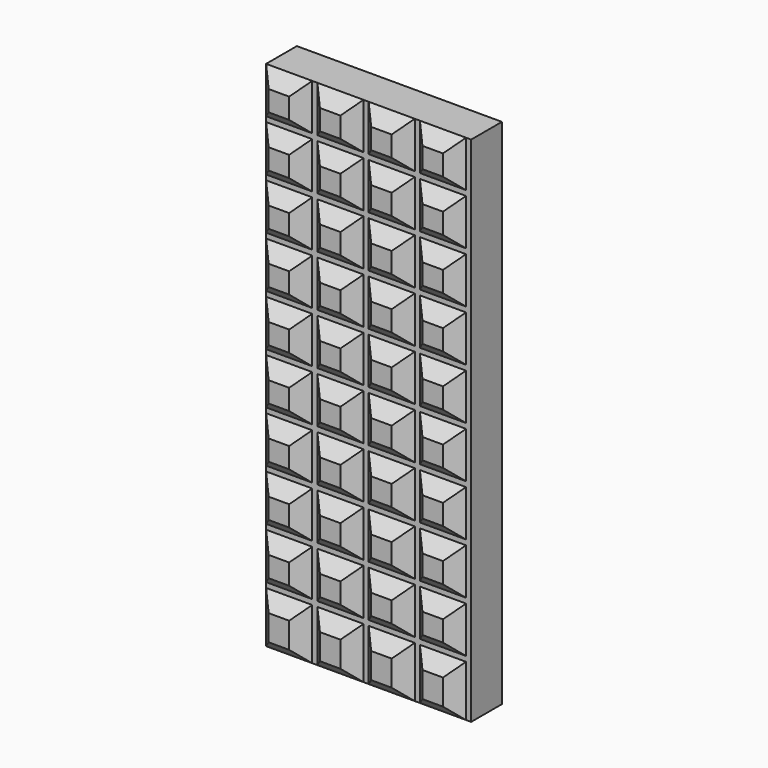
from build123d import *

# Parameters (mm, degrees)
F0_W     = 50.8
F0_H     = 127
F1_DEPTH = 12.7
F2_W     = 11.43
F2_H     = 11.43
F3_DEPTH = 3.175
F4_SIZE  = 3.17499


# Not quite as in the source:
# - a fillet or chamfer is up to 0.001 mm smaller than in the source, because OpenCascade refuses the exact size


with BuildPart() as f1:
    # F0 (on Front) → F1 (new body)
    with BuildSketch(Plane.XZ):
        with Locations((25.4, 63.5)):
            Rectangle(F0_W, F0_H)
    extrude(amount=F1_DEPTH)

    # F2 (on face) → F3 (cut)
    with BuildSketch(Plane.XZ.offset(12.7)):
        Polygon((11.43, 12.7), (11.43, 0), (12.7, 0), (12.7, 12.7), (24.13, 12.7), (24.13, 0), (25.4, 0), (25.4, 12.7), (36.83, 12.7), (36.83, 0), (38.1, 0), (38.1, 12.7), (49.53, 12.7), (49.53, 0), (50.8, 0), (50.8, 127), (49.53, 127), (49.53, 115.57), (38.1, 115.57), (38.1, 127), (36.83, 127), (36.83, 115.57), (25.4, 115.57), (25.4, 127), (24.13, 127), (24.13, 115.57), (12.7, 115.57), (12.7, 127), (11.43, 127), (11.43, 115.57), (0, 115.57), (0, 114.3), (11.43, 114.3), (11.43, 102.87), (0, 102.87), (0, 101.6), (11.43, 101.6), (11.43, 90.17), (0, 90.17), (0, 88.9), (11.43, 88.9), (11.43, 77.47), (0, 77.47), (0, 76.2), (11.43, 76.2), (11.43, 64.77), (0, 64.77), (0, 63.5), (11.43, 63.5), (11.43, 52.07), (0, 52.07), (0, 50.8), (11.43, 50.8), (11.43, 39.37), (0, 39.37), (0, 38.1), (11.43, 38.1), (11.43, 26.67), (0, 26.67), (0, 25.4), (11.43, 25.4), (11.43, 13.97), (0, 13.97), (0, 12.7), align=None)
        with Locations((18.415, 19.685)):
            Rectangle(F2_W, F2_H, mode=Mode.SUBTRACT)
        with Locations((18.415, 32.385)):
            Rectangle(F2_W, F2_H, mode=Mode.SUBTRACT)
        with Locations((18.415, 45.085)):
            Rectangle(F2_W, F2_H, mode=Mode.SUBTRACT)
        with Locations((18.415, 57.785)):
            Rectangle(F2_W, F2_H, mode=Mode.SUBTRACT)
        with Locations((31.115, 19.685)):
            Rectangle(F2_W, F2_H, mode=Mode.SUBTRACT)
        with Locations((43.815, 19.685)):
            Rectangle(F2_W, F2_H, mode=Mode.SUBTRACT)
        with Locations((31.115, 32.385)):
            Rectangle(F2_W, F2_H, mode=Mode.SUBTRACT)
        with Locations((31.115, 45.085)):
            Rectangle(F2_W, F2_H, mode=Mode.SUBTRACT)
        with Locations((31.115, 57.785)):
            Rectangle(F2_W, F2_H, mode=Mode.SUBTRACT)
        with Locations((43.815, 32.385)):
            Rectangle(F2_W, F2_H, mode=Mode.SUBTRACT)
        with Locations((43.815, 45.085)):
            Rectangle(F2_W, F2_H, mode=Mode.SUBTRACT)
        with Locations((43.815, 57.785)):
            Rectangle(F2_W, F2_H, mode=Mode.SUBTRACT)
        with Locations((18.415, 70.485)):
            Rectangle(F2_W, F2_H, mode=Mode.SUBTRACT)
        with Locations((18.415, 83.185)):
            Rectangle(F2_W, F2_H, mode=Mode.SUBTRACT)
        with Locations((18.415, 95.885)):
            Rectangle(F2_W, F2_H, mode=Mode.SUBTRACT)
        with Locations((18.415, 108.585)):
            Rectangle(F2_W, F2_H, mode=Mode.SUBTRACT)
        with Locations((31.115, 70.485)):
            Rectangle(F2_W, F2_H, mode=Mode.SUBTRACT)
        with Locations((31.115, 83.185)):
            Rectangle(F2_W, F2_H, mode=Mode.SUBTRACT)
        with Locations((43.815, 70.485)):
            Rectangle(F2_W, F2_H, mode=Mode.SUBTRACT)
        with Locations((43.815, 83.185)):
            Rectangle(F2_W, F2_H, mode=Mode.SUBTRACT)
        with Locations((31.115, 95.885)):
            Rectangle(F2_W, F2_H, mode=Mode.SUBTRACT)
        with Locations((31.115, 108.585)):
            Rectangle(F2_W, F2_H, mode=Mode.SUBTRACT)
        with Locations((43.815, 95.885)):
            Rectangle(F2_W, F2_H, mode=Mode.SUBTRACT)
        with Locations((43.815, 108.585)):
            Rectangle(F2_W, F2_H, mode=Mode.SUBTRACT)
    extrude(amount=-F3_DEPTH, mode=Mode.SUBTRACT)

    # F4 (size 3.175 in the source; OpenCascade refuses exactly that, so slightly less here)
    f4_edges = [f1.edges().sort_by_distance(p)[0] for p in [
        (11.43, -12.7, 6.35),
        (5.715, -12.7, 12.7),
        (18.415, -12.7, 12.7),
        (12.7, -12.7, 6.35),
        (24.13, -12.7, 6.35),
        (31.115, -12.7, 12.7),
        (25.4, -12.7, 6.35),
        (36.83, -12.7, 6.35),
        (38.1, -12.7, 6.35),
        (43.815, -12.7, 12.7),
        (43.815, -12.7, 13.97),
        (38.1, -12.7, 19.685),
        (43.815, -12.7, 25.4),
        (36.83, -12.7, 19.685),
        (12.7, -12.7, 19.685),
        (18.415, -12.7, 25.4),
        (24.13, -12.7, 19.685),
        (18.415, -12.7, 13.97),
        (25.4, -12.7, 32.385),
        (31.115, -12.7, 38.1),
        (36.83, -12.7, 32.385),
        (31.115, -12.7, 26.67),
        (12.7, -12.7, 32.385),
        (18.415, -12.7, 38.1),
        (24.13, -12.7, 32.385),
        (18.415, -12.7, 26.67),
        (31.115, -12.7, 25.4),
        (25.4, -12.7, 19.685),
        (31.115, -12.7, 13.97),
        (25.4, -12.7, 45.085),
        (31.115, -12.7, 50.8),
        (36.83, -12.7, 45.085),
        (31.115, -12.7, 39.37),
        (12.7, -12.7, 45.085),
        (18.415, -12.7, 50.8),
        (24.13, -12.7, 45.085),
        (18.415, -12.7, 39.37),
        (12.7, -12.7, 57.785),
        (18.415, -12.7, 63.5),
        (24.13, -12.7, 57.785),
        (18.415, -12.7, 52.07),
        (25.4, -12.7, 57.785),
        (31.115, -12.7, 63.5),
        (36.83, -12.7, 57.785),
        (31.115, -12.7, 52.07),
        (25.4, -12.7, 83.185),
        (31.115, -12.7, 88.9),
        (36.83, -12.7, 83.185),
        (31.115, -12.7, 77.47),
        (12.7, -12.7, 83.185),
        (18.415, -12.7, 88.9),
        (24.13, -12.7, 83.185),
        (18.415, -12.7, 77.47),
        (25.4, -12.7, 70.485),
        (31.115, -12.7, 76.2),
        (36.83, -12.7, 70.485),
        (31.115, -12.7, 64.77),
        (12.7, -12.7, 70.485),
        (18.415, -12.7, 76.2),
        (24.13, -12.7, 70.485),
        (18.415, -12.7, 64.77),
        (12.7, -12.7, 95.885),
        (18.415, -12.7, 101.6),
        (24.13, -12.7, 95.885),
        (18.415, -12.7, 90.17),
        (25.4, -12.7, 95.885),
        (31.115, -12.7, 101.6),
        (36.83, -12.7, 95.885),
        (31.115, -12.7, 90.17),
        (12.7, -12.7, 108.585),
        (18.415, -12.7, 114.3),
        (24.13, -12.7, 108.585),
        (18.415, -12.7, 102.87),
        (25.4, -12.7, 108.585),
        (31.115, -12.7, 114.3),
        (36.83, -12.7, 108.585),
        (31.115, -12.7, 102.87),
        (11.43, -12.7, 19.685),
        (5.715, -12.7, 25.4),
        (5.715, -12.7, 13.97),
        (5.715, -12.7, 26.67),
        (11.43, -12.7, 32.385),
        (5.715, -12.7, 38.1),
        (5.715, -12.7, 39.37),
        (11.43, -12.7, 45.085),
        (5.715, -12.7, 50.8),
        (5.715, -12.7, 52.07),
        (11.43, -12.7, 57.785),
        (5.715, -12.7, 63.5),
        (5.715, -12.7, 64.77),
        (11.43, -12.7, 70.485),
        (5.715, -12.7, 76.2),
        (5.715, -12.7, 77.47),
        (11.43, -12.7, 83.185),
        (5.715, -12.7, 88.9),
        (5.715, -12.7, 90.17),
        (11.43, -12.7, 95.885),
        (5.715, -12.7, 101.6),
        (5.715, -12.7, 114.3),
        (11.43, -12.7, 108.585),
        (5.715, -12.7, 102.87),
        (0, -12.7, 108.585),
        (5.715, -12.7, 127),
        (11.43, -12.7, 121.285),
        (5.715, -12.7, 115.57),
        (0, -12.7, 121.285),
        (18.415, -12.7, 127),
        (24.13, -12.7, 121.285),
        (18.415, -12.7, 115.57),
        (12.7, -12.7, 121.285),
        (31.115, -12.7, 127),
        (36.83, -12.7, 121.285),
        (31.115, -12.7, 115.57),
        (25.4, -12.7, 121.285),
        (43.815, -12.7, 127),
        (49.53, -12.7, 121.285),
        (43.815, -12.7, 115.57),
        (38.1, -12.7, 121.285),
        (38.1, -12.7, 108.585),
        (43.815, -12.7, 114.3),
        (49.53, -12.7, 108.585),
        (43.815, -12.7, 102.87),
        (38.1, -12.7, 95.885),
        (43.815, -12.7, 101.6),
        (49.53, -12.7, 95.885),
        (43.815, -12.7, 90.17),
        (38.1, -12.7, 83.185),
        (43.815, -12.7, 88.9),
        (49.53, -12.7, 83.185),
        (43.815, -12.7, 77.47),
        (38.1, -12.7, 70.485),
        (43.815, -12.7, 76.2),
        (49.53, -12.7, 70.485),
        (43.815, -12.7, 64.77),
        (0, -12.7, 95.885),
        (0, -12.7, 83.185),
        (0, -12.7, 70.485),
        (0, -12.7, 57.785),
        (38.1, -12.7, 45.085),
        (43.815, -12.7, 50.8),
        (49.53, -12.7, 45.085),
        (43.815, -12.7, 39.37),
        (38.1, -12.7, 32.385),
        (43.815, -12.7, 38.1),
        (49.53, -12.7, 32.385),
        (43.815, -12.7, 26.67),
        (49.53, -12.7, 19.685),
        (43.815, -12.7, 0),
        (49.53, -12.7, 6.35),
        (31.115, -12.7, 0),
        (18.415, -12.7, 0),
        (5.715, -12.7, 0),
        (0, -12.7, 6.35),
        (0, -12.7, 19.685),
        (0, -12.7, 32.385),
        (0, -12.7, 45.085),
        (38.1, -12.7, 57.785),
        (43.815, -12.7, 63.5),
        (49.53, -12.7, 57.785),
        (43.815, -12.7, 52.07),
    ]]
    chamfer(f4_edges, length=F4_SIZE)


solid = f1.part
